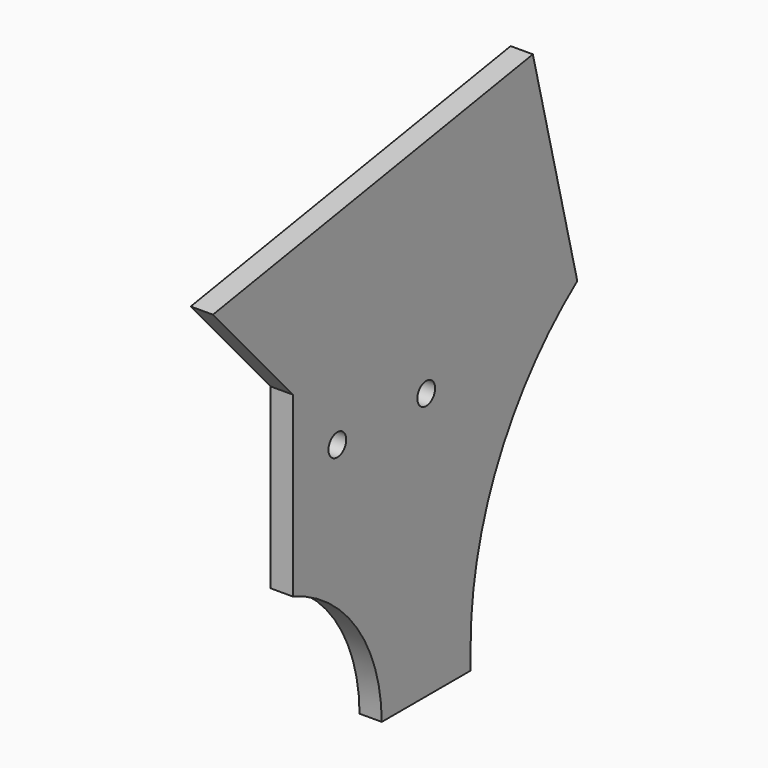
from build123d import *

# Parameters (mm, degrees)
F1_DEPTH    = 10
F3_D        = 10
F3_DEPTH    = 100
F3_TIP      = 3.0043030951
F5_DEPTH    = 25
F6_T1_DEPTH = 10


# Not quite as in the source:
# - a fillet or chamfer that OpenCascade refuses, or shapes differently, is made with other operations: its cross-section is extruded or revolved along the edge and cut away or added


with BuildPart() as f1:
    # F0 (on Right) → F1 (new body)
    with BuildSketch(Plane.YZ):
        Polygon((0, 150), (0, 0), (100, 0), (100, 100), (100, 200), (0, 200), align=None)
        Polygon((-45, 200), (0, 150), (0, 200), (100, 200), (100, 100), (160, 130), (135, 230), align=None)
    extrude(amount=F1_DEPTH)

    # F3
    with Locations(Plane.YZ.offset(10)):
        with Locations((25, 120), (75, 120)):
            Hole(F3_D / 2, depth=F3_DEPTH)
            with Locations((0, 0, -(F3_DEPTH + F3_TIP / 2))):  # 118° drill point
                Cone(0, F3_D / 2, F3_TIP, mode=Mode.SUBTRACT)

    # F4 (on face) → F5 (cut)
    with BuildSketch(Plane.YZ.offset(10)):
        with BuildLine():
            Line((0, 0), (50, 0))
            ThreePointArc((50, 0), (36.033388833, 42.8809920236), (0, 70))
            Line((0, 70), (0, 0))
        make_face()
    extrude(amount=-F5_DEPTH, mode=Mode.SUBTRACT)

    # F6: fillet of radius 150 on 1 edges, made by hand

    # F6_s2 → F6_t1 (join)
    with BuildSketch(Plane.YZ):
        with BuildLine():
            ThreePointArc((160, 130), (115.83592135, 77.082039325), (100, 10))
            Line((100, 10), (100, 100))
            Line((100, 100), (160, 130))
        make_face()
    extrude(amount=F6_T1_DEPTH)


solid = f1.part
